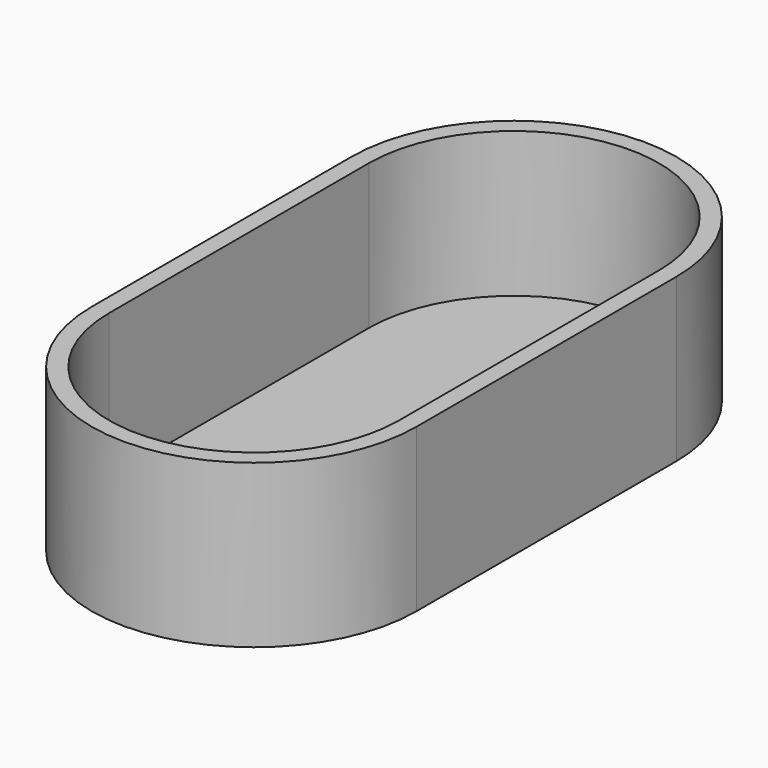
from build123d import *

# Parameters (mm, degrees)
F1_DEPTH = 15
F0_W     = 26.8
F0_H     = 30
F2_DEPTH = 1.6


# Not quite as in the source:
# - a feature names something its author has since deleted; it is built from what else it names


with BuildPart() as f1:
    # F0 (on Top) → F1 (new body)
    with BuildSketch(Plane.XY):
        with BuildLine():
            ThreePointArc((30, -15), (25.6066017178, -4.3933982822), (15, 0))
            ThreePointArc((15, 0), (4.3933982822, -4.3933982822), (0, -15))
            Line((0, -15), (0, -45))
            Line((0, -45), (1.6, -45))
            Line((1.6, -45), (1.6, -15))
            ThreePointArc((1.6, -15), (15, -1.6), (28.4, -15))
            Line((28.4, -15), (28.4, -45))
            Line((28.4, -45), (30, -45))
            Line((30, -45), (30, -15))
        make_face()
        with BuildLine():
            Line((1.6, -45), (0, -45))
            ThreePointArc((0, -45), (4.3933982822, -55.6066017178), (15, -60))
            ThreePointArc((15, -60), (25.6066017178, -55.6066017178), (30, -45))
            Line((30, -45), (28.4, -45))
            ThreePointArc((28.4, -45), (15, -58.4), (1.6, -45))
        make_face()
    extrude(amount=F1_DEPTH)

    # F0 (on Top) → F2 (join)
    with BuildSketch(Plane.XY):
        with BuildLine():
            ThreePointArc((28.4, -15), (15, -1.6), (1.6, -15))
            Line((1.6, -15), (28.4, -15))
        make_face()
        with BuildLine():
            Line((28.4, -45), (1.6, -45))
            ThreePointArc((1.6, -45), (15, -58.4), (28.4, -45))
        make_face()
        with Locations((15, -30)):
            Rectangle(F0_W, F0_H)
    extrude(amount=F2_DEPTH)


solid = f1.part
